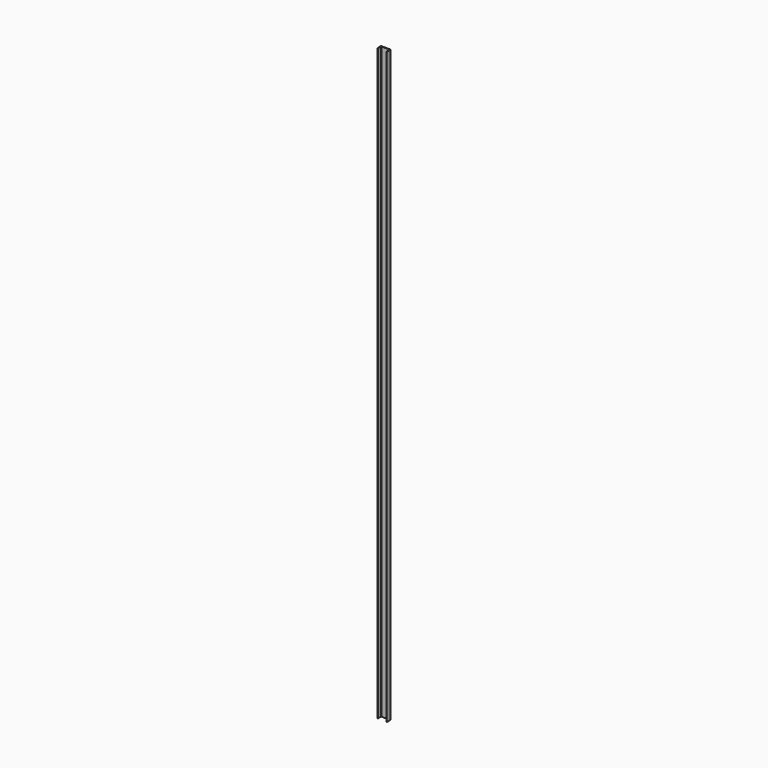
from build123d import *

# Parameters (mm, degrees)
F1_DEPTH    = 6000
F2_T1_DEPTH = 6000
F2_T3_DEPTH = 6025


# Not quite as in the source:
# - a fillet or chamfer that OpenCascade refuses, or shapes differently, is made with other operations: its cross-section is extruded or revolved along the edge and cut away or added


with BuildPart() as f1:
    # F0 (on Top) → F1 (new body)
    with BuildSketch(Plane.XY):
        Polygon((0, 50), (0, 0), (6, 0), (6, 44), (94, 44), (94, 0), (100, 0), (100, 50), align=None)
    extrude(amount=F1_DEPTH)

    # F2: fillet of radius 5 on 8 edges, made by hand

    # F2_s2 → F2_t1 (join)
    with BuildSketch(Plane.XY):
        with BuildLine():
            ThreePointArc((6, 39), (7.4644660941, 42.5355339059), (11, 44))
            Line((11, 44), (6, 44))
            Line((6, 44), (6, 39))
        make_face()
        with BuildLine():
            ThreePointArc((89, 44), (92.5355339059, 42.5355339059), (94, 39))
            Line((94, 39), (94, 44))
            Line((94, 44), (89, 44))
        make_face()
    extrude(amount=F2_T1_DEPTH)

    # F2_s4 → F2_t3 (cut)
    with BuildSketch(Plane.XY.offset(-12.5)):
        with BuildLine():
            ThreePointArc((1, 0), (4.5355339059, 1.4644660941), (6, 5))
            Line((6, 5), (6, 0))
            Line((6, 0), (1, 0))
        make_face()
        with BuildLine():
            ThreePointArc((0, 5), (1.4644660941, 1.4644660941), (5, 0))
            Line((5, 0), (0, 0))
            Line((0, 0), (0, 5))
        make_face()
        with BuildLine():
            ThreePointArc((100, 5), (98.5355339059, 1.4644660941), (95, 0))
            Line((95, 0), (100, 0))
            Line((100, 0), (100, 5))
        make_face()
        with BuildLine():
            ThreePointArc((94, 5), (95.4644660941, 1.4644660941), (99, 0))
            Line((99, 0), (94, 0))
            Line((94, 0), (94, 5))
        make_face()
        with BuildLine():
            ThreePointArc((0, 45), (1.4644660941, 48.5355339059), (5, 50))
            Line((5, 50), (0, 50))
            Line((0, 50), (0, 45))
        make_face()
        with BuildLine():
            ThreePointArc((95, 50), (98.5355339059, 48.5355339059), (100, 45))
            Line((100, 45), (100, 50))
            Line((100, 50), (95, 50))
        make_face()
    extrude(amount=F2_T3_DEPTH, mode=Mode.SUBTRACT)


solid = f1.part
